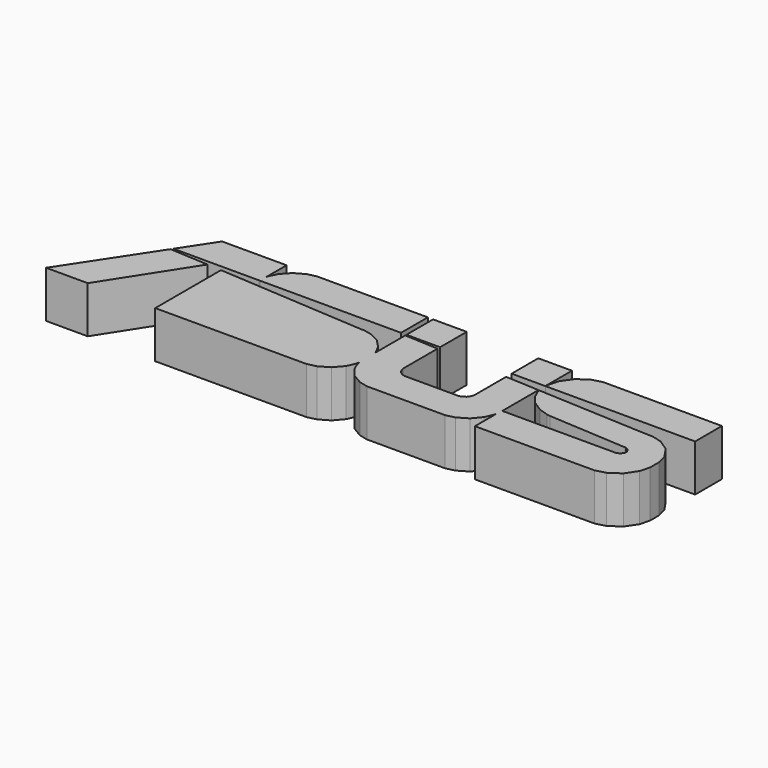
from build123d import *

# Parameters (mm, degrees)
F1_DEPTH = 5


# Not quite as in the source:
# - the program builds the solid bodies; features that only make, move or delete a surface that nothing else refers to are left out


with BuildPart() as f1:
    # F0 (on Top) → F1 (new body)
    with BuildSketch(Plane.XY):
        Polygon((1.633601, 6.434328), (1.582547, 6.434328), (-1.964563, 6.434328), (-1.964563, 2.873248), (1.633601, 2.873248), align=None)
    extrude(amount=F1_DEPTH)


with BuildPart() as f1b:
    # F0 (on Top) → F1, piece 2 (new body)
    with BuildSketch(Plane.XY):
        Polygon((-28.549473, -6.453378), (-22.858349, 2.415794), (-26.996771, 2.65557), (-33.000569, -6.453378), align=None)
    extrude(amount=F1_DEPTH)


with BuildPart() as f1c:
    # F0 (on Top) → F1, piece 3 (new body)
    with BuildSketch(Plane.XY):
        Polygon((12.915519, 2.873248), (28.884499, 2.871978), (28.884499, 6.451854), (16.559149, 6.451854), (16.207613, 6.451854), (15.157577, 6.171184), (14.005687, 5.403342), (13.220065, 4.266438), (12.921107, 3.22326), align=None)
    extrude(amount=F1_DEPTH)


with BuildPart() as f1d:
    # F0 (on Top) → F1, piece 4 (new body)
    with BuildSketch(Plane.XY):
        Polygon((9.277731, 6.434328), (9.277731, 2.873248), (12.877165, 2.873248), (12.877165, 6.434328), (9.329801, 6.434328), align=None)
    extrude(amount=F1_DEPTH)


with BuildPart() as f1e:
    # F0 (on Top) → F1, piece 5 (new body)
    with BuildSketch(Plane.XY):
        Polygon((12.877165, -2.871724), (12.817729, -3.543046), (12.817729, -6.453378), (25.238075, -6.453378), (25.590881, -6.453378), (26.653109, -6.165088), (27.812365, -5.381244), (28.596209, -4.221988), (28.884499, -3.15976), (28.884499, -2.807208), (28.884499, -2.290318), (28.884499, -1.935988), (28.596209, -0.873506), (27.812365, 0.285242), (26.653109, 1.06807), (25.590881, 1.354582), (25.238075, 1.354582), (24.557101, 1.385062), (23.589869, 1.427734), (13.943457, 1.898904), (12.979019, 1.948688), (13.034137, 1.671828), (13.384149, 0.87249), (14.130909, -0.039878), (15.197709, -0.719328), (16.211931, -1.050036), (16.559149, -1.096772), (24.973407, -1.613662), (25.083643, -1.613662), (25.417399, -1.796796), (25.603073, -2.130552), (25.603073, -2.242058), (25.603073, -2.352294), (25.417399, -2.685796), (25.083643, -2.871724), (24.973407, -2.871724), align=None)
        Polygon((-17.616297, -2.871978), (-17.616297, -2.871724), (-17.616297, 1.7653), (-17.616297, 2.08455006), (-21.338413, 2.327656), (-21.338413, -6.453378), (-17.912715, -6.453378), (-17.616297, -6.453378), align=None)
        Polygon((-1.964563, 2.72034), (-1.964563, -1.370838), (-1.911985, -3.50139), (-1.861185, -3.801872), (-1.490599, -4.66725), (-0.711835, -5.602986), (0.339725, -6.225794), (1.271143, -6.453378), (1.582547, -6.453378), (9.329801, -6.453378), (9.637141, -6.453378), (10.561701, -6.230112), (11.607927, -5.615432), (12.386437, -4.691888), (12.762357, -3.838956), (12.817729, -3.543046), (12.877165, -2.871724), (12.877165, 1.954022), (9.277731, 2.140204), (9.277731, -1.986788), (9.277731, -2.08915), (9.194927, -2.394966), (8.969121, -2.729738), (8.635365, -2.954528), (8.329549, -3.038602), (8.227441, -3.038602), (2.683637, -3.038602), (2.581529, -3.038602), (2.275713, -2.954528), (1.940941, -2.729738), (1.716151, -2.394966), (1.633601, -2.08915), (1.633601, -1.986788), (1.633601, 2.534412), align=None)
        Polygon((-17.616297, 1.7653), (-17.616297, -2.871724), (-17.616297, -2.871978), (-17.616297, -6.453378), (-5.491099, -6.453378), (-5.176647, -6.453378), (-4.232529, -6.227318), (-3.161919, -5.60578), (-2.361565, -4.668774), (-1.971421, -3.803396), (-1.911985, -3.50139), (-1.964563, -1.370838), (-2.038985, -1.091184), (-2.452243, -0.301752), (-3.250057, 0.541528), (-4.286631, 1.094232), (-5.190363, 1.292606), (-5.491099, 1.292606), (-17.616297, 2.08455006), align=None)
    extrude(amount=F1_DEPTH)


with BuildPart() as f1f:
    # F0 (on Top) → F1, piece 6 (new body)
    with BuildSketch(Plane.XY):
        Polygon((-17.616297, 2.8732391208), (-2.536571, 2.871978), (-2.536571, 6.451854), (-14.077569, 6.451854), (-14.382115, 6.451854), (-15.294229, 6.242812), (-16.338931, 5.662422), (-17.138015, 4.784598), (-17.546193, 3.97002), (-17.616297, 3.682238), align=None)
        Polygon((-17.722469, 2.873248), (-17.616297, 2.8732391208), (-17.616297, 3.682238), (-17.616297, 6.434328), (-24.505031, 6.434328), (-26.853007, 2.873248), align=None)
    extrude(amount=F1_DEPTH)


solid = Compound([f1.part, f1b.part, f1c.part, f1d.part, f1e.part, f1f.part])
